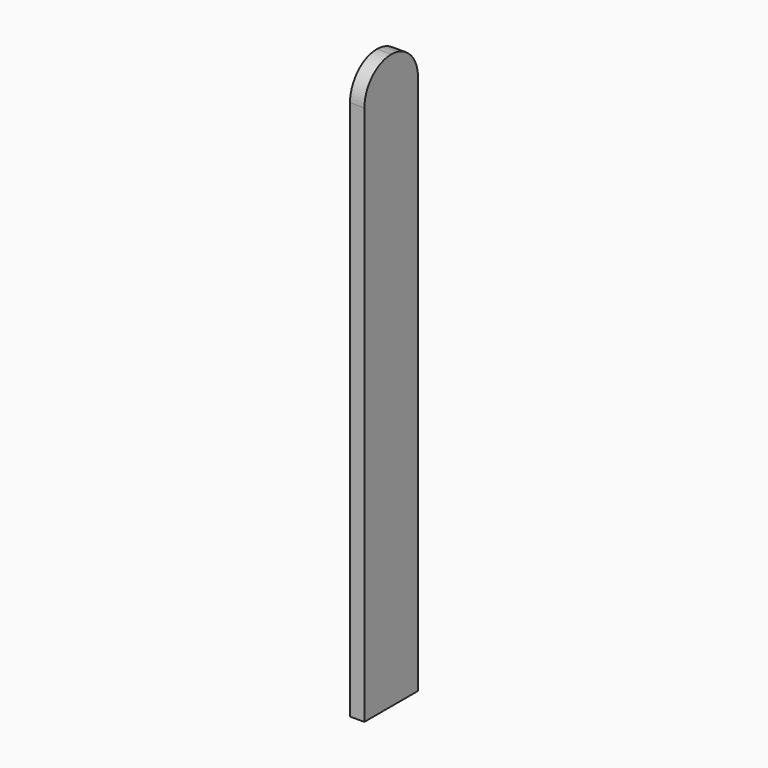
from build123d import *

# Parameters (mm, degrees)
F0_W     = 88.9
F0_H     = 762
F1_DEPTH = 19.05
F2_R     = 44.44999


# Not quite as in the source:
# - a fillet or chamfer is up to 0.001 mm smaller than in the source, because OpenCascade refuses the exact size


with BuildPart() as f1:
    # F0 (on Right) → F1 (new body)
    with BuildSketch(Plane.YZ):
        with Locations((44.45, 381)):
            Rectangle(F0_W, F0_H)
    extrude(amount=F1_DEPTH)

    # F2 (radius 44.45 in the source; OpenCascade refuses exactly that, so slightly less here)
    f2_edges = [f1.edges().sort_by_distance(p)[0] for p in [
        (9.525, 0, 762),
        (9.525, 88.9, 762),
    ]]
    fillet(f2_edges, radius=F2_R)


solid = f1.part
